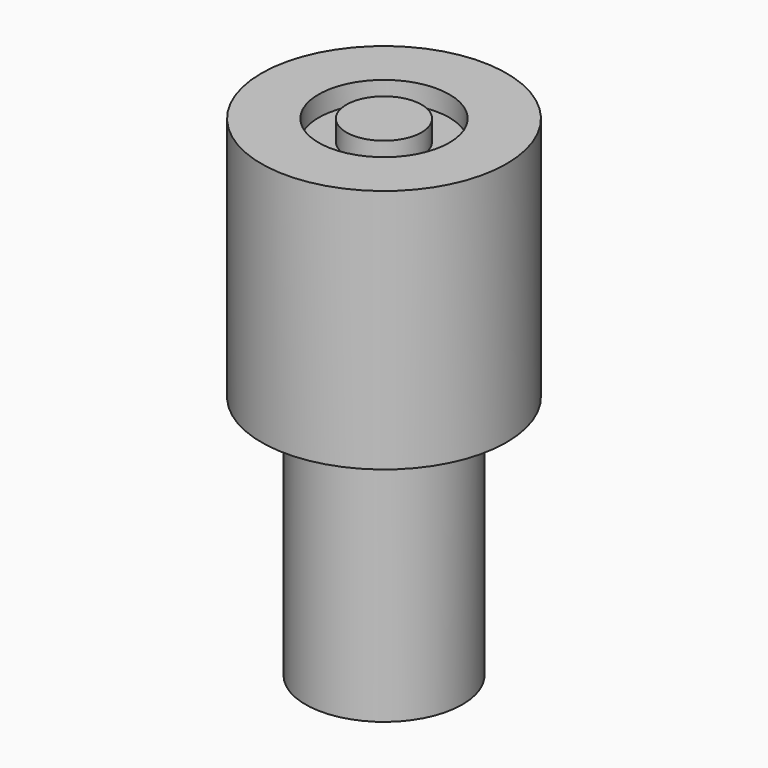
from build123d import *

# Parameters (mm, degrees)
F0_R     = 3.048
F1_DEPTH = 4.7625
F2_R     = 4.7625
F3_DEPTH = 9.525
F4_R     = 2.54
F4_R_2   = 1.4605
F5_DEPTH = 0.79375


# Not quite as in the source:
# - a length typed as a fraction of an inch, garbled in the dataset ("3 / 203.2 mm" for 3/8 in), is restored


with BuildPart() as f1:
    # F0 (on Top) → F1 (new body, symmetric)
    with BuildSketch(Plane.XY):
        Circle(F0_R)
    extrude(amount=F1_DEPTH, both=True)

    # F2 (on face) → F3 (join)
    with BuildSketch(Plane.XY.offset(4.7625)):
        Circle(F2_R)
    extrude(amount=F3_DEPTH)

    # F4 (on face) → F5 (cut)
    with BuildSketch(Plane.XY.offset(14.2875)):
        Circle(F4_R)
        Circle(F4_R_2, mode=Mode.SUBTRACT)
    extrude(amount=-F5_DEPTH, mode=Mode.SUBTRACT)


solid = f1.part
